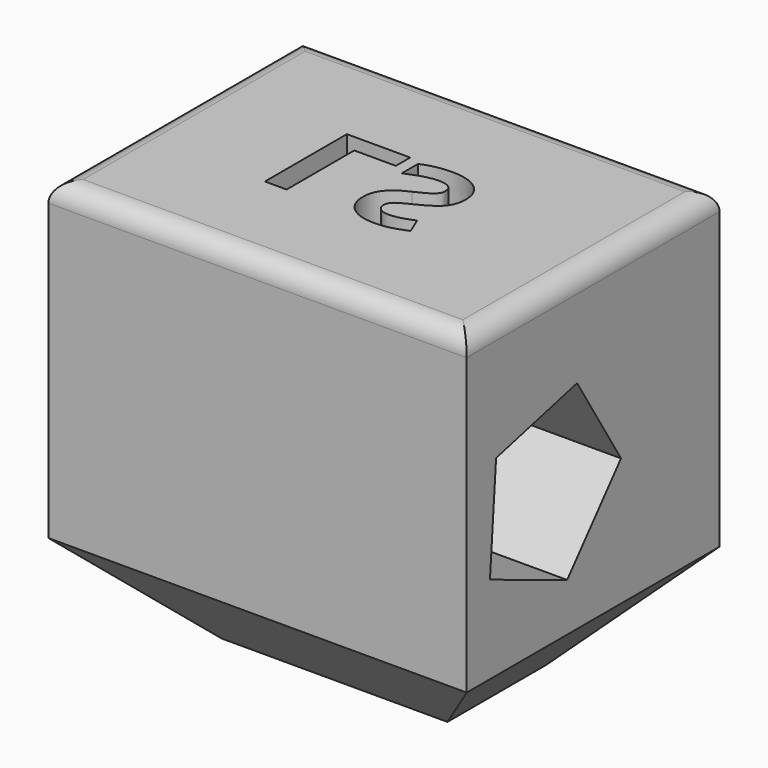
from build123d import *

# Parameters (mm, degrees)
F0_W         = 110.3667020798
F0_H         = 83.3917055279
F1_DEPTH     = 108.2730386406
F2_R         = 5.08
F3_TEXT_SIZE = 37.8840344234
F4_DEPTH     = 254
F5_SIZE      = 25.4
F7_DEPTH     = 127


# Not quite as in the source:
# - Text() gives the source's letters only with a copy of the font that has no kerning and outlines rounded to 1/6400 em; it was checked with that copy


with BuildPart() as f1:
    # F0 (on Top) → F1 (new body)
    with BuildSketch(Plane.XY):
        with Locations((2.2454634309, 14.1488490626)):
            Rectangle(F0_W, F0_H)
    extrude(amount=F1_DEPTH)

    # F2
    f2_edges = [f1.edges().sort_by_distance(p)[0] for p in [
        (2.245463, -27.547004, 108.273039),
        (2.245463, 55.844702, 108.273039),
        (57.428814, 14.148849, 108.273039),
        (-52.937888, 14.148849, 108.273039),
    ]]
    fillet(f2_edges, radius=F2_R)

    # F3 (on face) → F4 (cut)
    with BuildSketch(Plane(origin=(0, 0, 0), x_dir=(1, 0, 0), z_dir=(0, 0, -1))):
        with Locations((-21.4563328773, -27.2765047848)):
            Text('LS', F3_TEXT_SIZE, font='Open Sans', font_style=FontStyle.BOLD, text_align=(TextAlign.LEFT, TextAlign.BOTTOM))
    extrude(amount=-F4_DEPTH, mode=Mode.SUBTRACT)

    # F5
    f5_edges = [f1.edges().sort_by_distance(p)[0] for p in [
        (57.428814, 14.148849, 0),
        (2.245463, 55.844702, 0),
        (2.245463, -27.547004, 0),
        (-52.937888, 14.148849, 0),
    ]]
    chamfer(f5_edges, length=F5_SIZE)

    # F6 (on face) → F7 (cut)
    with BuildSketch(Plane.YZ.offset(57.4288144708)):
        Polygon((23.3361373579, 59.108889542), (8.8465002442, 82.4909444233), (-17.8686995256, 75.9359329492), (-19.8899638857, 48.5026581803), (5.5760258092, 38.1029734245), align=None)
    extrude(amount=-F7_DEPTH, mode=Mode.SUBTRACT)


solid = f1.part
